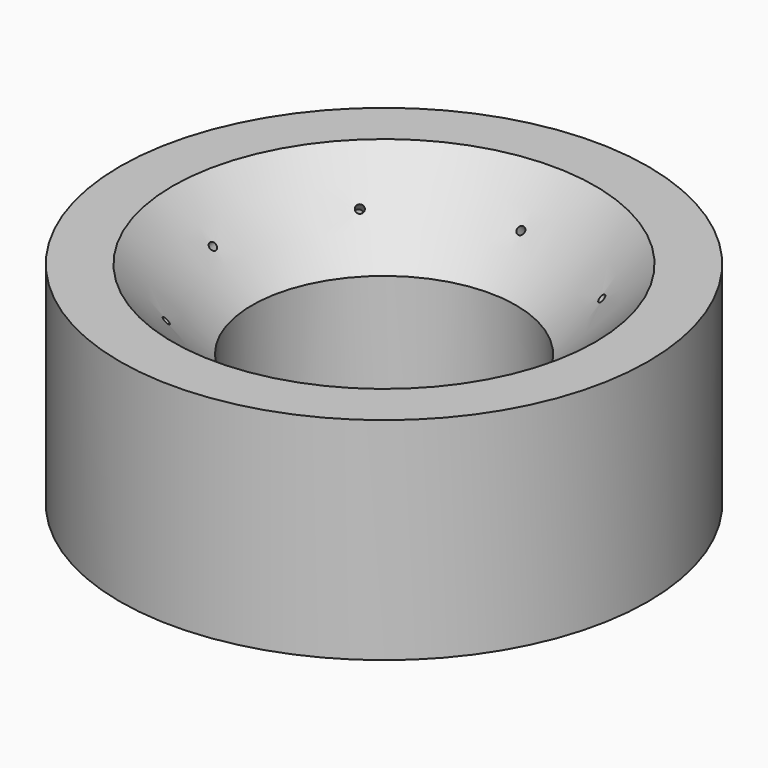
from build123d import *

# Parameters (mm, degrees)
F0_R      = 50
F1_DEPTH  = 40
F2_R      = 25
F3_DEPTH  = 50
F5_SIZE   = 15
F6_T      = -2.5
F10_R     = 0.75
F11_DEPTH = 15
F13_COUNT = 8


with BuildPart() as f1:
    # F0 (on Top) → F1 (new body)
    with BuildSketch(Plane.XY):
        Circle(F0_R)
    extrude(amount=F1_DEPTH)

    # F2 (on face) → F3 (cut)
    with BuildSketch(Plane(origin=(0, 0, 0), x_dir=(1, 0, 0), z_dir=(0, 0, -1))):
        Circle(F2_R)
    extrude(amount=-F3_DEPTH, mode=Mode.SUBTRACT)

    # F5
    f5_edges = [f1.edges().sort_by_distance(p)[0] for p in [
        (-25, 0, 40),
    ]]
    chamfer(f5_edges, length=F5_SIZE)

    # F6
    f6_openings = [f1.faces().sort_by_distance(p)[0] for p in [
        (-48.585786, 0, 0),
    ]]
    offset(amount=F6_T, openings=f6_openings)

    # F10 (on line) → F11 (cut, symmetric)
    with BuildSketch(Plane(origin=(0, -0.6375, 0.6375), x_dir=(-1, 0, 0), z_dir=(0, 0.7071067812, -0.7071067812))):
        with Locations((0, 45.8103796311)):
            Circle(F10_R)
    f11 = extrude(amount=F11_DEPTH, both=True, mode=Mode.SUBTRACT)

    # F13: F11 ×8 about axis
    f13_axis = Axis((0, 0, 54.5265711844), (0, 0, 1))
    for i in range(1, F13_COUNT):
        add(f11.rotate(f13_axis, i * 360 / F13_COUNT), mode=Mode.SUBTRACT)


solid = f1.part
